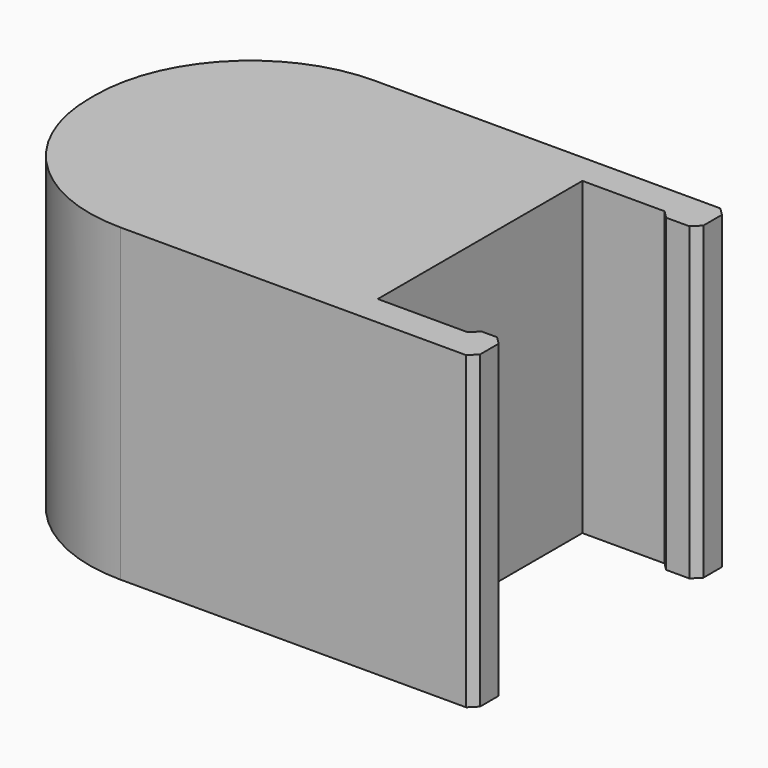
from build123d import *

# Parameters (mm, degrees)
F0_W     = 5.8
F0_H     = 2
F1_DEPTH = 20
F2_R     = 10
F3_SIZE  = 0.49999


# Not quite as in the source:
# - a fillet or chamfer is up to 0.001 mm smaller than in the source, because OpenCascade refuses the exact size


with BuildPart() as f1:
    # F0 (on Top) → F1 (new body)
    with BuildSketch(Plane.XY):
        with Locations((-39.9097009659, 46.350823313)):
            Rectangle(F0_W, F0_H)
        Polygon((-42.8097009659, 45.350823313), (-42.8097009659, 47.350823313), (-67.8097009659, 47.350823313), (-67.8097009659, 26.850823313), (-42.8097009659, 26.850823313), (-42.8097009659, 28.850823313), align=None)
        Polygon((-35.0097009659, 47.350823313), (-37.0097009659, 47.350823313), (-37.0097009659, 45.350823313), (-37.0097009659, 44.850823313), (-35.0097009659, 44.850823313), align=None)
        with Locations((-39.9097009659, 27.850823313)):
            Rectangle(F0_W, F0_H)
        Polygon((-37.0097009659, 29.350823313), (-37.0097009659, 28.850823313), (-37.0097009659, 26.850823313), (-35.0097009659, 26.850823313), (-35.0097009659, 29.350823313), align=None)
    extrude(amount=F1_DEPTH)

    # F2
    f2_edges = [f1.edges().sort_by_distance(p)[0] for p in [
        (-67.809701, 47.350823, 10),
        (-67.809701, 26.850823, 10),
    ]]
    fillet(f2_edges, radius=F2_R)

    # F3 (size 0.5 in the source; OpenCascade refuses exactly that, so slightly less here)
    f3_edges = [f1.edges().sort_by_distance(p)[0] for p in [
        (-35.009701, 47.350823, 10),
        (-35.009701, 44.850823, 10),
        (-35.009701, 29.350823, 10),
        (-35.009701, 26.850823, 10),
        (-37.009701, 29.350823, 10),
        (-37.009701, 45.350823, 10),
    ]]
    chamfer(f3_edges, length=F3_SIZE)


solid = f1.part
